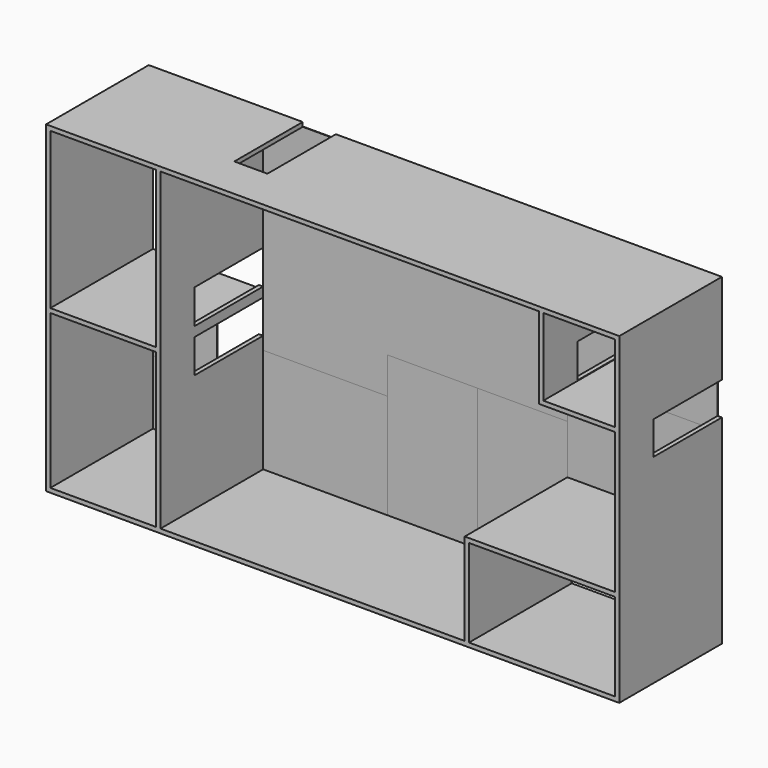
from build123d import *

# Parameters (mm, degrees)
F0_W      = 9194.8
F0_H      = 7670.8
F0_W_2    = 8991.6
F0_H_2    = 7467.6
F1_DEPTH  = 3048
F2_W      = 3048
F2_H      = 101.6
F3_DEPTH  = 1701.8
F4_W      = 3048
F4_H      = 5530.85
F5_DEPTH  = 2336.8
F6_W      = 101.6
F6_H      = 3048
F7_DEPTH  = 7670.8
F8_W      = 3048
F8_H      = 101.6
F9_DEPTH  = 1701.8
F10_W     = 3048
F10_H     = 101.6
F11_DEPTH = 3568.7
F12_W     = 101.6
F12_H     = 3048
F13_DEPTH = 2082.8
F14_W     = 3048
F14_H     = 101.6
F15_DEPTH = 2514.6
F16_W     = 101.6
F16_H     = 3048
F17_DEPTH = 7670.8
F18_W     = 787.4
F18_H     = 2032
F19_DEPTH = 5664.2
F20_W     = 2032
F20_H     = 812.8
F20_H_2   = 800.1
F21_DEPTH = 2133.6
F22_W     = 2032
F22_H     = 812.8
F23_DEPTH = 355.6
F24_W     = 2032
F24_H     = 787.4
F25_DEPTH = 2870.2
F27_DEPTH = 12.7
F28_W     = 2870.2
F28_H     = 1936.75
F29_DEPTH = 12.7
F30_W     = 2870.2
F30_H     = 1936.75
F31_DEPTH = 12.7
F32_W     = 3568.7
F32_H     = 2127.2500000001
F33_DEPTH = 12.7
F34_W     = 1524
F34_H     = 2133.6
F35_DEPTH = 12.7
F36_W     = 2514.6
F36_H     = 1524
F37_DEPTH = 12.7
F38_W     = 2959.1
F38_H     = 2489.2
F39_DEPTH = 12.7
F40_DEPTH = 12.7
F41_DEPTH = 12.7
F42_W     = 6007.1
F42_H     = 958.85
F43_DEPTH = 12.7
F44_W     = 1739.9
F44_H     = 863.6
F45_DEPTH = 12.7


with BuildPart() as f1:
    # F0 (on Front) → F1 (new body)
    with BuildSketch(Plane.XZ):
        with Locations((-7169.6171020508, -428.8149536133)):
            Rectangle(F0_W, F0_H)
        with Locations((-7169.6171020508, -428.8149536133)):
            Rectangle(F0_W_2, F0_H_2, mode=Mode.SUBTRACT)
    extrude(amount=F1_DEPTH)

    # F2 (on face) → F3 (join)
    with BuildSketch(Plane.YZ.offset(-2572.2171020508)):
        with Locations((-1524, 3355.7850463867)):
            Rectangle(F2_W, F2_H)
        with Locations((-1524, 1419.0350463867)):
            Rectangle(F2_W, F2_H)
    extrude(amount=F3_DEPTH)

    # F4 (on face) → F5 (cut)
    with BuildSketch(Plane.YZ.offset(-2572.2171020508)):
        with Locations((-1524, -1397.1899536133)):
            Rectangle(F4_W, F4_H)
    extrude(amount=-F5_DEPTH, mode=Mode.SUBTRACT)

    # F6 (on face) → F7 (join, through all)
    with BuildSketch(Plane.XY.offset(3406.5850463867)):
        with Locations((-819.6171020508, -1524)):
            Rectangle(F6_W, F6_H)
    extrude(amount=-F7_DEPTH)

    # F8 (on face) → F9 (join, through all)
    with BuildSketch(Plane.YZ.offset(-2572.2171020508)):
        with Locations((-1524, -4213.4149536133)):
            Rectangle(F8_W, F8_H)
    extrude(amount=F9_DEPTH)

    # F10 (on face) → F11 (join)
    with BuildSketch(Plane(origin=(-870.4171020508, 0, 0), x_dir=(0, -1, 0), z_dir=(-1, 0, 0))):
        with Locations((1524, -2029.0149536133)):
            Rectangle(F10_W, F10_H)
    extrude(amount=F11_DEPTH)

    # F12 (on face) → F13 (join, through all)
    with BuildSketch(Plane(origin=(0, 0, -2079.8149536133), x_dir=(1, 0, 0), z_dir=(0, 0, -1))):
        with Locations((-4388.3171020508, 1524)):
            Rectangle(F12_W, F12_H)
    extrude(amount=F13_DEPTH)

    # F14 (on face) → F15 (join)
    with BuildSketch(Plane(origin=(-11767.0171020508, 0, 0), x_dir=(0, -1, 0), z_dir=(-1, 0, 0))):
        with Locations((1524, 3355.7850463867)):
            Rectangle(F14_W, F14_H)
        with Locations((1524, -4213.4149536133)):
            Rectangle(F14_W, F14_H)
        with Locations((1524, -454.2149536133)):
            Rectangle(F14_W, F14_H)
    extrude(amount=F15_DEPTH)

    # F16 (on face) → F17 (join, through all)
    with BuildSketch(Plane(origin=(0, 0, -4264.2149536133), x_dir=(1, 0, 0), z_dir=(0, 0, -1))):
        with Locations((-14332.4171020508, 1524)):
            Rectangle(F16_W, F16_H)
    extrude(amount=-F17_DEPTH)

    # F18 (on face) → F19 (cut)
    with BuildSketch(Plane(origin=(0, 0, 3304.9850463867), x_dir=(1, 0, 0), z_dir=(0, 0, -1))):
        with Locations((-10331.9171020508, 1016)):
            Rectangle(F18_W, F18_H)
    extrude(amount=-F19_DEPTH, mode=Mode.SUBTRACT)

    # F20 (on face) → F21 (cut)
    with BuildSketch(Plane(origin=(-11767.0171020508, 0, 0), x_dir=(0, -1, 0), z_dir=(-1, 0, 0))):
        with Locations((1016, 66.4850463867)):
            Rectangle(F20_W, F20_H)
        with Locations((1016, -968.5649536133)):
            Rectangle(F20_W, F20_H_2)
    extrude(amount=-F21_DEPTH, mode=Mode.SUBTRACT)

    # F22 (on face) → F23 (cut)
    with BuildSketch(Plane(origin=(-2673.8171020508, 0, 0), x_dir=(0, -1, 0), z_dir=(-1, 0, 0))):
        with Locations((1016, 1888.9350463867)):
            Rectangle(F22_W, F22_H)
    extrude(amount=-F23_DEPTH, mode=Mode.SUBTRACT)

    # F24 (on face) → F25 (cut)
    with BuildSketch(Plane(origin=(-870.4171020508, 0, 0), x_dir=(0, -1, 0), z_dir=(-1, 0, 0))):
        with Locations((1016, 860.2350463867)):
            Rectangle(F24_W, F24_H)
    extrude(amount=-F25_DEPTH, mode=Mode.SUBTRACT)


with BuildPart() as f27:
    # F26 (on face) → F27 (new body)
    with BuildSketch(Plane(origin=(0, 0, 0), x_dir=(-1, 0, 0), z_dir=(0, 1, 0))):
        Polygon((3893.0171020508, 1368.2350463867), (3893.0171020508, 3304.9850463867), (2673.8171020508, 3304.9850463867), (2673.8171020508, 1368.2350463867), (870.4171020508, 1368.2350463867), (870.4171020508, 149.0350463867), (10446.2171020508, 149.0350463867), (10446.2171020508, -1673.4149536133), (11665.4171020508, -1673.4149536133), (11665.4171020508, 3304.9850463867), (9633.4171020508, 3304.9850463867), (9633.4171020508, 1368.2350463867), align=None)
    extrude(amount=F27_DEPTH)

    # F42 (on face) + F27_face (on face) → F43 (join, through all)
    with BuildSketch(Plane.XZ):
        with Locations((-7442.6671020508, -330.3899536133)):
            Rectangle(F42_W, F42_H)
    with BuildSketch(Plane(origin=(-7228.9160188464, 0, 1061.078645363), x_dir=(-1, 0, 0), z_dir=(0, -1, 0))):
        Polygon((-3335.8989167956, -307.1564010237), (2404.5010832044, -307.1564010237), (2404.5010832044, -2243.9064010237), (4436.5010832044, -2243.9064010237), (4436.5010832044, 2734.4935989763), (3217.3010832044, 2734.4935989763), (3217.3010832044, 912.0435989763), (-6358.4989167956, 912.0435989763), (-6358.4989167956, -307.1564010234), (-4555.0989167956, -307.1564010237), (-4555.0989167956, -2243.9064010237), (-3335.8989167956, -2243.9064010237), align=None)
    extrude(amount=-F43_DEPTH)

    # F44 (on face) → F45 (join, through all)
    with BuildSketch(Plane.XZ):
        with Locations((-9576.2671020508, -1241.6149536133)):
            Rectangle(F44_W, F44_H)
    extrude(amount=-F45_DEPTH)


with BuildPart() as f29:
    # F28 (on face) → F29 (new body, through all)
    with BuildSketch(Plane.XZ):
        with Locations((-8198.3171020508, 2336.6100463867)):
            Rectangle(F28_W, F28_H)
    extrude(amount=-F29_DEPTH)


with BuildPart() as f31:
    # F30 (on face) → F31 (new body)
    with BuildSketch(Plane.XZ):
        with Locations((-5328.1171020508, 2336.6100463867)):
            Rectangle(F30_W, F30_H)
    extrude(amount=-F31_DEPTH)


with BuildPart() as f33:
    # F32 (on face) → F33 (new body)
    with BuildSketch(Plane.XZ):
        with Locations((-2654.7671020508, -914.5899536133)):
            Rectangle(F32_W, F32_H)
    extrude(amount=-F33_DEPTH)


with BuildPart() as f35:
    # F34 (on face) → F35 (new body)
    with BuildSketch(Plane.XZ):
        with Locations((-13519.6171020508, -1571.8149536133)):
            Rectangle(F34_W, F34_H)
    extrude(amount=-F35_DEPTH)


with BuildPart() as f37:
    # F36 (on face) → F37 (new body)
    with BuildSketch(Plane.XZ):
        with Locations((-13024.3171020508, -3400.6149536133)):
            Rectangle(F36_W, F36_H)
    extrude(amount=-F37_DEPTH)


with BuildPart() as f39:
    # F38 (on face) → F39 (new body)
    with BuildSketch(Plane.XZ):
        with Locations((-10185.8671020508, -2918.0149536133)):
            Rectangle(F38_W, F38_H)
    extrude(amount=-F39_DEPTH)


with BuildPart() as f40:
    # F38 (on face) → F40 (new body)
    with BuildSketch(Plane.XZ):
        Polygon((-6572.7171020508, -4162.6149536133), (-6572.7171020508, -809.8149536133), (-8706.3171020508, -809.8149536133), (-8706.3171020508, -1673.4149536133), (-8706.3171020508, -4162.6149536133), align=None)
    extrude(amount=-F40_DEPTH)


with BuildPart() as f41:
    # F38 (on face) → F41 (new body)
    with BuildSketch(Plane.XZ):
        Polygon((-4439.1171020508, -809.8149536133), (-6572.7171020508, -809.8149536133), (-6572.7171020508, -4162.6149536133), (-4439.1171020508, -4162.6149536133), (-4439.1171020508, -1978.2149536134), align=None)
    extrude(amount=-F41_DEPTH)


solid = Compound([f1.part, f27.part, f29.part, f31.part, f33.part, f35.part, f37.part, f39.part, f40.part, f41.part])
